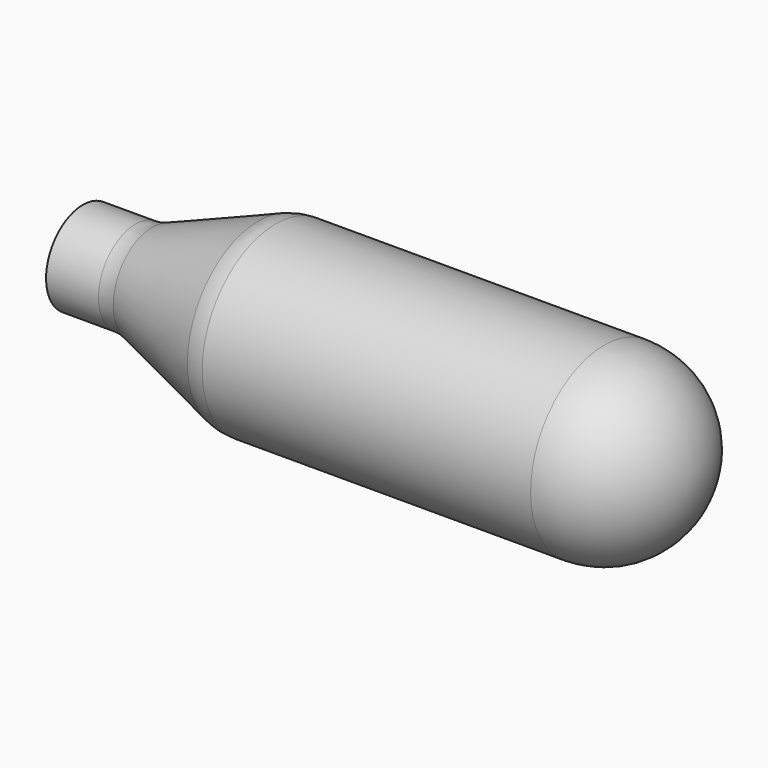
from build123d import *

# Parameters (mm, degrees)
F2_R = 9.525
F3_R = 5.08


# Not quite as in the source:
# - a feature of the source that left no trace in its solid (it failed there, or was rolled back) is left out


with BuildPart() as f1:
    # F0 (on Front) → F1 (revolve)
    with BuildSketch(Plane.XZ):
        Polygon((0, 4.7625), (0, 0), (63.5, 0), (63.5, 9.525), (19.05, 9.525), (6.35, 4.7625), (4.6010445803, 4.7625), align=None)
    revolve(axis=Axis((31.75, 0, 0), (1, 0, 0)))

    # F2
    f2_edges = [f1.edges().sort_by_distance(p)[0] for p in [
        (63.5, 0, -9.525),
    ]]
    fillet(f2_edges, radius=F2_R)

    # F3
    f3_edges = [f1.edges().sort_by_distance(p)[0] for p in [
        (19.05, 0, -9.525),
        (6.35, 0, -4.7625),
    ]]
    fillet(f3_edges, radius=F3_R)


solid = f1.part
